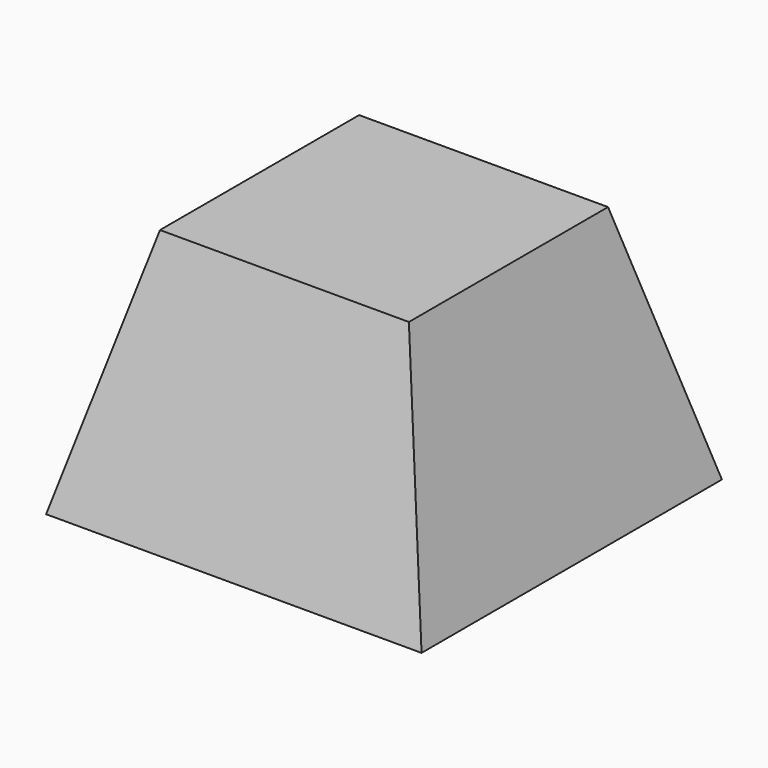
from build123d import *

# Parameters (mm, degrees)
F0_W        = 300
F0_H        = 193.6492
F1_DEPTH    = 300
F2_T1_DEPTH = 1338.777968426
F2_T3_DEPTH = 1338.777968426


# Not quite as in the source:
# - a fillet or chamfer that OpenCascade refuses, or shapes differently, is made with other operations: its cross-section is extruded or revolved along the edge and cut away or added


with BuildPart() as f1:
    # F0 (on Front) → F1 (new body)
    with BuildSketch(Plane.XZ):
        with Locations((1.8808934838, -61.8465812054)):
            Rectangle(F0_W, F0_H)
    extrude(amount=F1_DEPTH)

    # F2: chamfer of 200 x 51.6397698104 on 4 edges, made by hand

    # F2_s2 → F2_t1 (cut)
    with BuildSketch(Plane.XZ.offset(-519.388984213)):
        Polygon((100.2411236733, 34.9780187946), (151.8808934838, -165.0219812054), (151.8808934838, 34.9780187946), align=None)
        Polygon((-96.4793367058, 34.9780187946), (-148.1191065162, -165.0219812054), (-148.1191065162, 34.9780187946), align=None)
    extrude(amount=F2_T1_DEPTH, mode=Mode.SUBTRACT)

    # F2_s4 → F2_t3 (cut)
    with BuildSketch(Plane.YZ.offset(-667.5080907292)):
        Polygon((-51.6397698104, 34.9780187946), (0, -165.0219812054), (0, 34.9780187946), align=None)
        Polygon((-248.3602301896, 34.9780187946), (-300, -165.0219812054), (-300, 34.9780187946), align=None)
    extrude(amount=F2_T3_DEPTH, mode=Mode.SUBTRACT)


solid = f1.part
